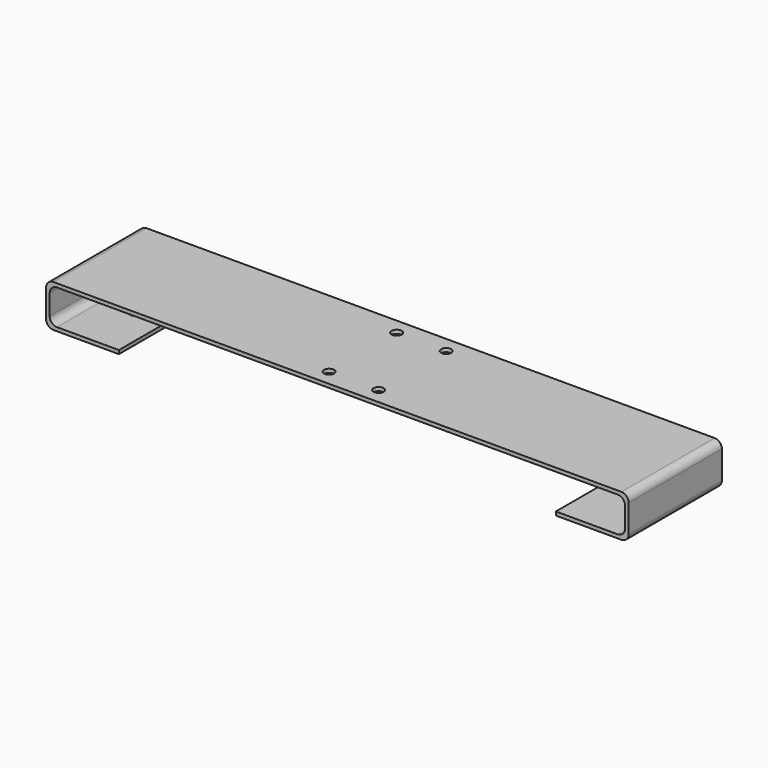
from build123d import *

# Parameters (mm, degrees)
F1_DEPTH = 40
F4_D     = 9
F4_DEPTH = 12
F4_TIP   = 2.7038727856
F5_D     = 9
F5_DEPTH = 12
F5_TIP   = 2.7038727856
F7_D     = 7
F8_R     = 5


# Not quite as in the source:
# - a feature names something its author has since deleted; it is built from what else it names


with BuildPart() as f1:
    # F0 (on Front) → F1 (new body, symmetric)
    with BuildSketch(Plane.XZ):
        Polygon((0, 29), (0, 0), (50, 0), (50, 2.5), (2.5, 2.5), (2.5, 26.5), (397.5, 26.5), (397.5, 2.5), (350, 2.5), (350, 0), (400, 0), (400, 29), align=None)
    extrude(amount=F1_DEPTH, both=True)

    # F4 (one way)
    with BuildSketch(Plane.XY.offset(2.5)):
        with Locations((370, 0)):
            Circle(F4_D / 2)
    extrude(amount=-F4_DEPTH, mode=Mode.SUBTRACT)
    with Locations(Plane.XY.offset(2.5)):
        with Locations((370, 0)):
            with Locations((0, 0, -(F4_DEPTH + F4_TIP / 2))):  # 118° drill point
                Cone(0, F4_D / 2, F4_TIP, mode=Mode.SUBTRACT)

    # F5 (one way)
    with BuildSketch(Plane.XY.offset(2.5)):
        with Locations((30, 0)):
            Circle(F5_D / 2)
    extrude(amount=-F5_DEPTH, mode=Mode.SUBTRACT)
    with Locations(Plane.XY.offset(2.5)):
        with Locations((30, 0)):
            with Locations((0, 0, -(F5_DEPTH + F5_TIP / 2))):  # 118° drill point
                Cone(0, F5_D / 2, F5_TIP, mode=Mode.SUBTRACT)

    # F7 (through all)
    with Locations(Plane(origin=(0, 0, 26.5), x_dir=(1, 0, 0), z_dir=(0, 0, -1))):
        with Locations((219.5, -29), (185.5, -29), (185.5, 29), (219.5, 29)):
            Hole(F7_D / 2)

    # F8
    f8_edges = [f1.edges().sort_by_distance(p)[0] for p in [
        (0, 0, 29),
        (0, 0, 0),
        (400, 0, 29),
        (400, 0, 0),
        (2.5, 0, 2.5),
        (2.5, 0, 26.5),
        (397.5, 0, 2.5),
        (397.5, 0, 26.5),
    ]]
    fillet(f8_edges, radius=F8_R)


solid = f1.part
